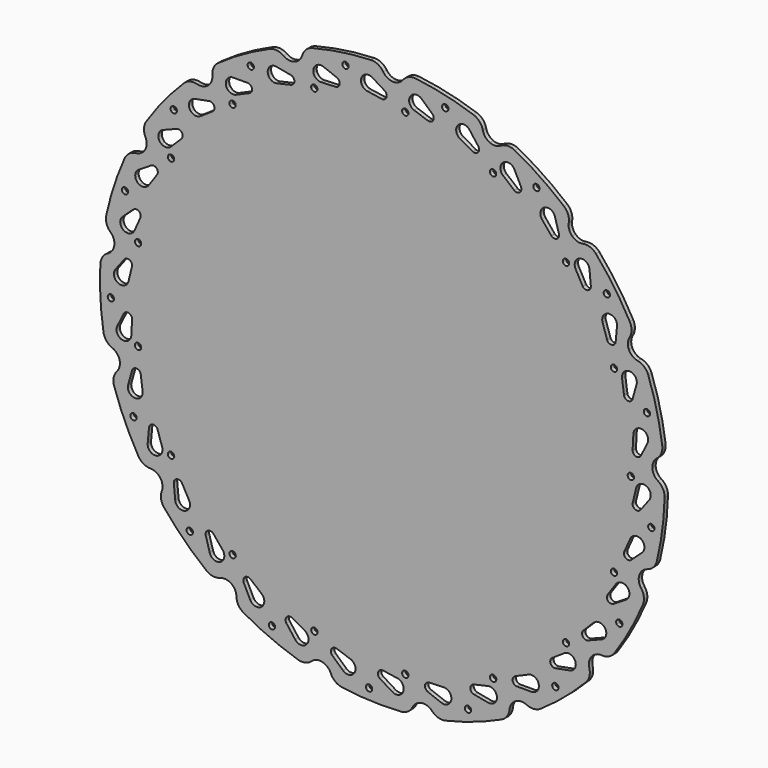
from build123d import *

# Parameters (mm, degrees)
F0_R            = 101.6
F1_DEPTH        = 1.524
F3_DEPTH        = 1.525
F3_COPIES_COUNT = 34
F5_DEPTH        = 1.525
F5_COPIES_COUNT = 17
F6_R            = 5.08


# Not quite as in the source:
# - a pattern or mirror of a feature is missing from the dataset's text; its kind, count and spacing are read off the source's solid


with BuildPart() as f1:
    # F0 (on Front) → F1 (new body)
    with BuildSketch(Plane.XZ):
        Circle(F0_R)
    extrude(amount=F1_DEPTH)

    # F2 (on face) → F3 (cut, through all)
    with BuildSketch(Plane(origin=(0, 0, 0), x_dir=(-1, 0, 0), z_dir=(0, 1, 0))):
        with BuildLine():
            ThreePointArc((5.3984134663, 91.2073362022), (7.0300665956, 92.1022261773), (7.6793204393, 93.8462415007))
            ThreePointArc((7.6793204393, 93.8462415007), (6.3118932421, 96.1751896603), (3.6118292281, 96.1159360545))
            ThreePointArc((3.6118292281, 96.1159360545), (2.4930857864, 94.7216532688), (2.5061602196, 92.9340737785))
            ThreePointArc((2.5061602196, 92.9340737785), (3.6451785704, 91.5563043596), (5.3984134663, 91.2073362022))
        make_face()
        with BuildLine():
            ThreePointArc((2.5061602196, 92.9340737785), (2.4930857864, 94.7216532688), (3.6118292281, 96.1159360545))
            Line((3.6118292281, 96.1159360545), (-0.8336257209, 93.3729147192))
            ThreePointArc((-0.8336257209, 93.3729147192), (0.5210784334, 93.5214504925), (1.4917620355, 92.5648630338))
            Line((1.4917620355, 92.5648630338), (2.5061602196, 92.9340737785))
        make_face()
        with BuildLine():
            Line((0.229817278, 90.4511290928), (5.3984134663, 91.2073362022))
            ThreePointArc((5.3984134663, 91.2073362022), (3.6451785704, 91.5563043596), (2.5061602196, 92.9340737785))
            Line((2.5061602196, 92.9340737785), (1.4917620355, 92.5648630338))
            ThreePointArc((1.4917620355, 92.5648630338), (1.5633823079, 92.2975725383), (1.5875, 92.0219060562))
            ThreePointArc((1.5875, 92.0219060562), (1.2010393788, 90.983801697), (0.229817278, 90.4511290928))
        make_face()
        with BuildLine():
            ThreePointArc((1.4917620355, 92.5648630338), (0.5210784334, 93.5214504925), (-0.8336257209, 93.3729147192))
            ThreePointArc((-0.8336257209, 93.3729147192), (-1.5272332013, 91.5886451663), (0, 90.4344060562))
            Line((0, 90.4344060562), (0, 92.0219060562))
            Line((0, 92.0219060562), (1.4917620355, 92.5648630338))
        make_face()
        with BuildLine():
            ThreePointArc((0, 90.4344060562), (0.1152124572, 90.438592335), (0.229817278, 90.4511290928))
            ThreePointArc((0.229817278, 90.4511290928), (1.2010393788, 90.983801697), (1.5875, 92.0219060562))
            ThreePointArc((1.5875, 92.0219060562), (1.5633823079, 92.2975725383), (1.4917620355, 92.5648630338))
            Line((1.4917620355, 92.5648630338), (0, 92.0219060562))
            Line((0, 92.0219060562), (0, 90.4344060562))
        make_face()
    f3 = extrude(amount=-F3_DEPTH, mode=Mode.SUBTRACT)

    # F3_copies: F3 ×34 about axis
    f3_copies_axis = Axis((0, 0, 0), (0, 1, 0))
    for i in range(1, F3_COPIES_COUNT):
        add(f3.rotate(f3_copies_axis, i * 360 / F3_COPIES_COUNT), mode=Mode.SUBTRACT)

    # F4 (on face) → F5 (cut, through all)
    with BuildSketch(Plane(origin=(0, 0, 0), x_dir=(-1, 0, 0), z_dir=(0, 1, 0))):
        with BuildLine():
            ThreePointArc((0.3524865069, 101.5225822304), (-7.0778161141, 104.5156903801), (-3.7969791697, 97.2078724856))
            ThreePointArc((-3.7969791697, 97.2078724856), (-0.8532108722, 98.5294740808), (0.3524865069, 101.5225822304))
        make_face()
        with BuildLine():
            ThreePointArc((14.3898468752, 96.8433640167), (13.0483670081, 97.9689992784), (12.1727782097, 96.4524349929))
            ThreePointArc((12.1727782097, 96.4524349929), (13.4453267423, 95.717728755), (14.3898468752, 96.8433640167))
        make_face()
        with BuildLine():
            ThreePointArc((-7.0915264359, 89.0247835403), (-7.1088911743, 89.2232634073), (-7.1604577704, 89.4157125641))
            ThreePointArc((-7.1604577704, 89.4157125641), (-9.3601616976, 88.8263036732), (-7.0915264359, 89.0247835403))
        make_face()
    f5 = extrude(amount=-F5_DEPTH, mode=Mode.SUBTRACT)

    # F5_copies: F5 ×17 about axis
    f5_copies_axis = Axis((0, 0, 0), (0, 1, 0))
    for i in range(1, F5_COPIES_COUNT):
        add(f5.rotate(f5_copies_axis, i * 360 / F5_COPIES_COUNT), mode=Mode.SUBTRACT)

    # F6
    f6_edges = [f1.edges().sort_by_distance(p)[0] for p in [
        (8.275668, -0.762, 101.262398),
        (-0.351803, -0.762, 101.599391),
        (-28.863367, -0.762, 97.41389),
        (36.373886, -0.762, 94.865697),
        (44.297028, -0.762, 91.434858),
        (68.187081, -0.762, 75.319864),
        (74.335829, -0.762, 69.258534),
        (90.791233, -0.762, 45.601667),
        (94.335164, -0.762, 37.728461),
        (101.133526, -0.762, 9.724712),
        (101.594013, -0.762, 1.10295),
        (97.817175, -0.762, -27.46562),
        (95.132028, -0.762, -35.67152),
        (81.290073, -0.762, -60.946567),
        (75.821934, -0.762, -67.628354),
        (53.784296, -0.762, -86.196343),
        (46.271669, -0.762, -90.451604),
        (19.014652, -0.762, -99.804825),
        (10.472158, -0.762, -101.058864),
        (-18.323026, -0.762, -99.934112),
        (-26.741676, -0.762, -98.017564),
        (-53.186078, -0.762, -86.566744),
        (-60.343898, -0.762, -81.738449),
        (-80.866055, -0.762, -61.508057),
        (-85.796342, -0.762, -54.420103),
        (-97.624624, -0.762, -28.142367),
        (-99.661515, -0.762, -19.752021),
        (-101.198446, -0.762, 9.024107),
        (-100.066849, -0.762, 17.58368),
        (-91.104857, -0.762, 44.971824),
        (-86.957599, -0.762, 52.544609),
        (-68.707053, -0.762, 74.845848),
        (-62.104245, -0.762, 80.409097),
        (-37.02998, -0.762, 94.611525),
    ]]
    fillet(f6_edges, radius=F6_R)


solid = f1.part
